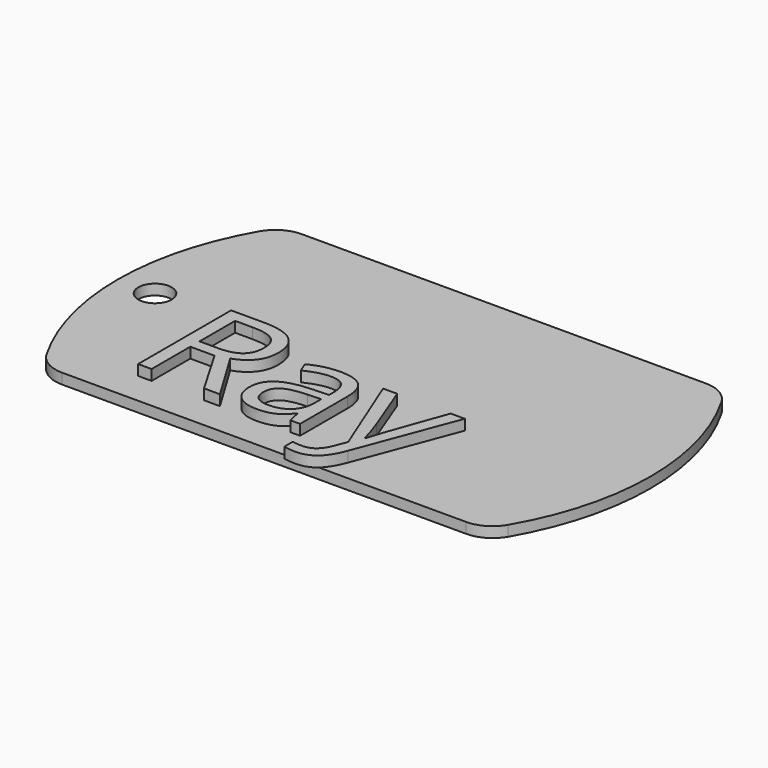
from build123d import *

# Parameters (mm, degrees)
F1_DEPTH     = 1
F3_R         = 1.5875
F4_DEPTH     = 1
F5_TEXT_SIZE = 15.5083938605
F6_DEPTH     = 1


# Not quite as in the source:
# - Text() gives the source's letters only with a copy of the font that has no kerning and outlines rounded to 1/6400 em; it was checked with that copy


with BuildPart() as f1:
    # F0 (on Top) → F1 (new body)
    with BuildSketch(Plane.XY):
        with BuildLine():
            ThreePointArc((-19.2474145991, 14.2875), (-20.8349145991, 13.862130657), (-21.9970452561, 12.7))
            ThreePointArc((-21.9970452561, 12.7), (-25.4, 0), (-21.9970452561, -12.7))
            ThreePointArc((-21.9970452561, -12.7), (-20.8349145991, -13.862130657), (-19.2474145991, -14.2875))
            Line((-19.2474145991, -14.2875), (19.2474145991, -14.2875))
            ThreePointArc((19.2474145991, -14.2875), (20.8349145991, -13.862130657), (21.9970452561, -12.7))
            ThreePointArc((21.9970452561, -12.7), (25.4, 0), (21.9970452561, 12.7))
            ThreePointArc((21.9970452561, 12.7), (20.8349145991, 13.862130657), (19.2474145991, 14.2875))
            Line((19.2474145991, 14.2875), (-19.2474145991, 14.2875))
        make_face()
    extrude(amount=F1_DEPTH)

    # F3 (on face) → F4 (cut)
    with BuildSketch(Plane.XY.offset(1)):
        with Locations((-21.821282804, 0)):
            Circle(F3_R)
    extrude(amount=-F4_DEPTH, mode=Mode.SUBTRACT)

    # F5 (on face) → F6 (join)
    with BuildSketch(Plane.XY.offset(1)):
        with Locations((-16.0189960152, -11.1660435796)):
            Text('Ray', F5_TEXT_SIZE, font='Open Sans', text_align=(TextAlign.LEFT, TextAlign.BOTTOM))
    extrude(amount=F6_DEPTH)


solid = f1.part
